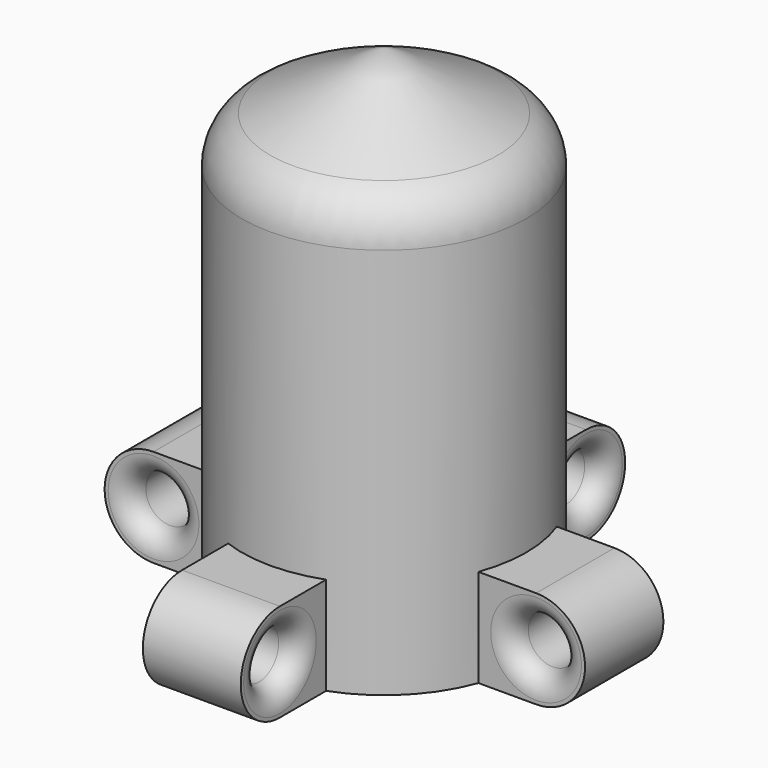
from build123d import *

# Parameters (mm, degrees)
F0_R            = 13.843
F0_R_2          = 10.668
F1_DEPTH        = 38.1
F2_R            = 2.38125
F3_DEPTH        = 4.7625
F3_COPIES_COUNT = 4
F4_R            = 2.032


# Not quite as in the source:
# - a pattern or mirror of a feature is missing from the dataset's text; its kind, count and spacing are read off the source's solid


with BuildPart() as f1:
    # F0 (on Top) → F1 (new body)
    with BuildSketch(Plane.XY):
        Circle(F0_R)
        Circle(F0_R_2, mode=Mode.SUBTRACT)
    extrude(amount=F1_DEPTH)

    # F2 (on Front) → F3 (join, symmetric)
    with BuildSketch(Plane.XZ):
        with BuildLine():
            ThreePointArc((18.6055, 0), (13.843, 4.7625), (18.6055, 9.525))
            Line((18.6055, 9.525), (13.843, 9.525))
            Line((13.843, 9.525), (11.303, 9.525))
            Line((11.303, 9.525), (11.303, 0))
            Line((11.303, 0), (13.843, 0))
            Line((13.843, 0), (18.6055, 0))
        make_face()
        with BuildLine():
            ThreePointArc((18.6055, 0), (21.9730960454, 1.3949039546), (23.368, 4.7625))
            ThreePointArc((23.368, 4.7625), (21.9730960454, 8.1300960454), (18.6055, 9.525))
            ThreePointArc((18.6055, 9.525), (13.843, 4.7625), (18.6055, 0))
        make_face()
        with Locations((18.6055, 4.7625)):
            Circle(F2_R, mode=Mode.SUBTRACT)
    f3 = extrude(amount=F3_DEPTH, both=True)

    # F3_copies: F3 ×4 about axis
    f3_copies_axis = Axis((0, 0, 0), (0, 0, 1))
    for i in range(1, F3_COPIES_COUNT):
        add(f3.rotate(f3_copies_axis, i * 360 / F3_COPIES_COUNT))

    # F4
    f4_edges = [f1.edges().sort_by_distance(p)[0] for p in [
        (16.22425, -4.7625, 4.7625),
        (16.22425, 4.7625, 4.7625),
        (-16.22425, -4.7625, 4.7625),
        (-16.22425, 4.7625, 4.7625),
        (-4.7625, 16.22425, 4.7625),
        (4.7625, 16.22425, 4.7625),
        (-4.7625, -16.22425, 4.7625),
        (4.7625, -16.22425, 4.7625),
    ]]
    fillet(f4_edges, radius=F4_R)

    # F5 (on Front) → F6 (revolve)
    with BuildSketch(Plane.XZ):
        with BuildLine():
            Line((0, 48.26), (-11.0671968277, 42.6273697639))
            ThreePointArc((-11.0671968277, 42.6273697639), (-13.0938036139, 40.7552853063), (-13.843, 38.1))
            Line((-13.843, 38.1), (-10.668, 38.1))
            ThreePointArc((-10.668, 38.1), (-10.2156632287, 39.7031620073), (-8.9920738104, 40.8334566201))
            Line((-8.9920738104, 40.8334566201), (0, 45.4099566696))
            Line((0, 45.4099566696), (0, 48.26))
        make_face()
    revolve(axis=Axis((0, 0, 0), (0, 0, -1)))


solid = f1.part
